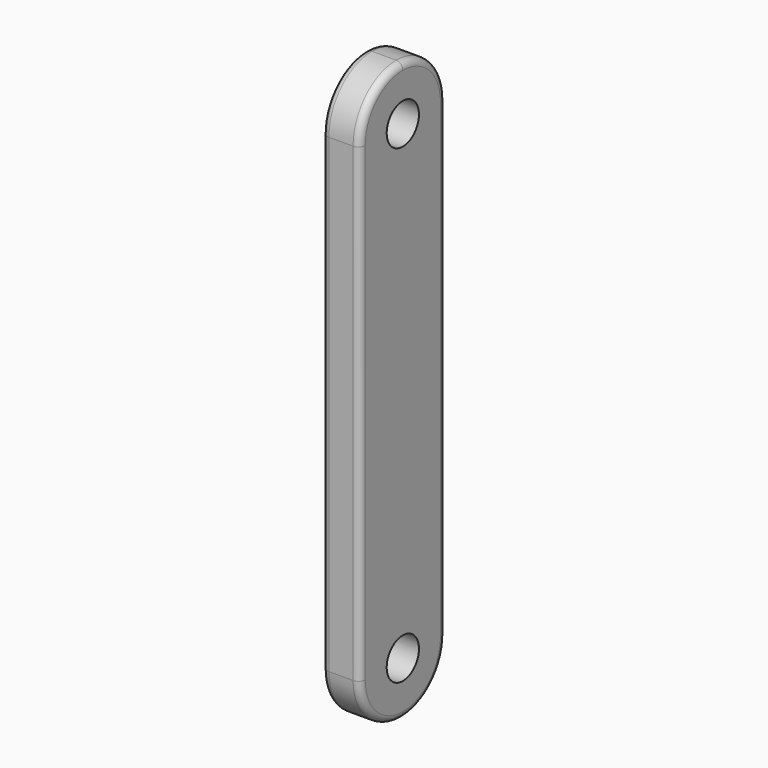
from build123d import *

# Parameters (mm, degrees)
F0_W     = 2.8
F0_H     = 8
F1_DEPTH = 43
F2_R     = 3.99999
F3_R     = 1.5
F4_DEPTH = 5
F5_R     = 0.5


# Not quite as in the source:
# - a fillet or chamfer is up to 0.001 mm smaller than in the source, because OpenCascade refuses the exact size


with BuildPart() as f1:
    # F0 (on Top) → F1 (new body)
    with BuildSketch(Plane.XY):
        Rectangle(F0_W, F0_H)
    extrude(amount=F1_DEPTH)

    # F2 (radius 4 in the source; OpenCascade refuses exactly that, so slightly less here)
    f2_edges = [f1.edges().sort_by_distance(p)[0] for p in [
        (0, 4, 0),
        (0, -4, 0),
        (0, -4, 43),
        (0, 4, 43),
    ]]
    fillet(f2_edges, radius=F2_R)

    # F3 (on face) → F4 (cut)
    with BuildSketch(Plane(origin=(-1.4, 0, 0), x_dir=(0, -1, 0), z_dir=(-1, 0, 0))):
        with Locations((0, 4)):
            Circle(F3_R)
        with Locations((0, 39)):
            Circle(F3_R)
    extrude(amount=-F4_DEPTH, mode=Mode.SUBTRACT)

    # F5
    f5_edges = [f1.edges().sort_by_distance(p)[0] for p in [
        (-1.4, 4, 21.5),
        (1.4, 4, 21.5),
    ]]
    fillet(f5_edges, radius=F5_R)


solid = f1.part
